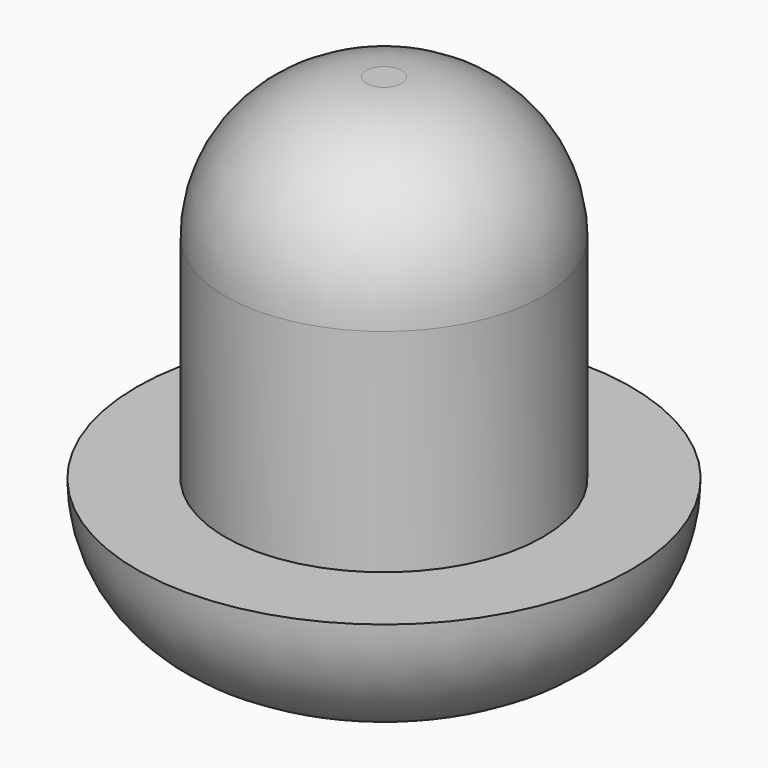
from build123d import *

# Parameters (mm, degrees)
F0_R     = 3.5
F0_R_2   = 2.25
F1_DEPTH = 2
F2_DEPTH = 5
F3_R     = 1.99999


# Not quite as in the source:
# - a fillet or chamfer is up to 0.001 mm smaller than in the source, because OpenCascade refuses the exact size


with BuildPart() as f1:
    # F0 (on Top) → F1 (new body)
    with BuildSketch(Plane.XY):
        Circle(F0_R)
        Circle(F0_R_2, mode=Mode.SUBTRACT)
        Circle(F0_R_2)
    extrude(amount=-F1_DEPTH)

    # F0 (on Top) → F2 (join)
    with BuildSketch(Plane.XY):
        Circle(F0_R_2)
    extrude(amount=F2_DEPTH)

    # F3 (radius 2 in the source; OpenCascade refuses exactly that, so slightly less here)
    f3_edges = [f1.edges().sort_by_distance(p)[0] for p in [
        (-2.25, 0, 5),
        (-3.5, 0, -2),
    ]]
    fillet(f3_edges, radius=F3_R)


solid = f1.part
